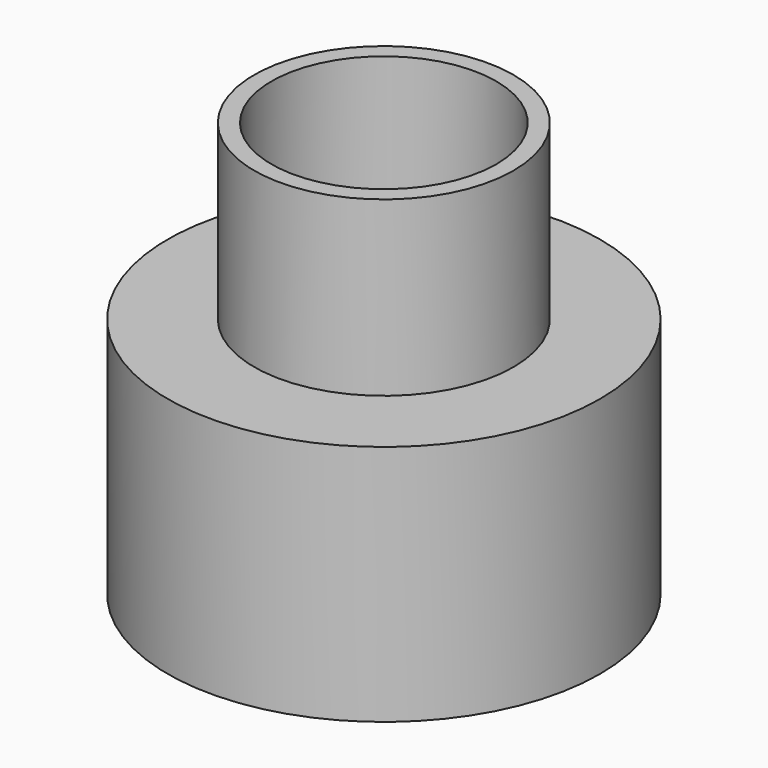
from build123d import *

# Parameters (mm, degrees)
F0_R     = 31.75
F0_R_2   = 8.3458742529
F1_DEPTH = 38.1
F2_T     = -2.54
F3_R     = 19.05
F3_R_2   = 8.3458742529
F4_DEPTH = 25.4
F6_T     = -2.54


# Not quite as in the source:
# - a fillet or chamfer that OpenCascade refuses, or shapes differently, is made with other operations: its cross-section is extruded or revolved along the edge and cut away or added
# - the program builds the solid bodies; features that only make, move or delete a surface that nothing else refers to are left out


with BuildPart() as f1:
    # F0 (on Top) → F1 (new body)
    with BuildSketch(Plane.XY):
        Circle(F0_R)
        Circle(F0_R_2, mode=Mode.SUBTRACT)
    extrude(amount=F1_DEPTH)

    # F2
    f2_openings = [f1.faces().sort_by_distance(p)[0] for p in [
        (-30.851974, 0, 0),
        (-8.345874, 0, 19.05),
    ]]
    offset(amount=F2_T, openings=f2_openings)

    # F3 (on face) → F4 (join)
    with BuildSketch(Plane.XY.offset(38.1)):
        Circle(F3_R)
        Circle(F3_R_2, mode=Mode.SUBTRACT)
    extrude(amount=F4_DEPTH)

    # F6
    f6_openings = [f1.faces().sort_by_distance(p)[0] for p in [
        (-18.511185, 0, 63.5),
        (-8.345874, 0, 49.53),
    ]]
    offset(amount=F6_T, openings=f6_openings, kind=Kind.INTERSECTION)

    # F7: chamfer of 5.08 on 1 edges, made by hand

    # F7_s1 → F7_t2 (revolve, cut)
    with BuildSketch(Plane.XZ):
        Polygon((34.29, 0), (29.21, 5.08), (29.21, 0), align=None)
    revolve(axis=Axis((0, 0, 0), (0, 0, 1)), mode=Mode.SUBTRACT)


solid = f1.part
